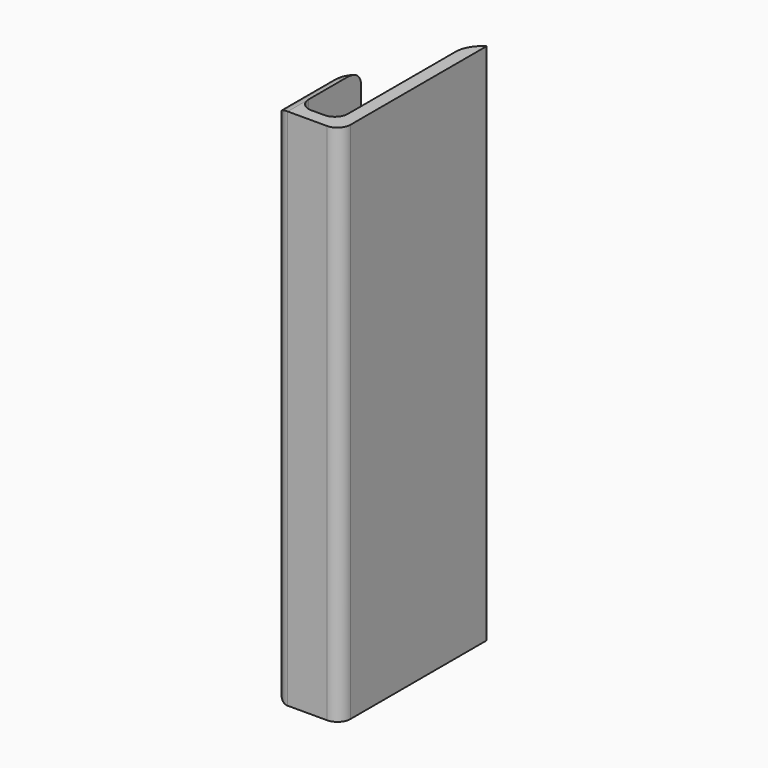
from build123d import *

# Parameters (mm, degrees)
F1_DEPTH    = 40
F2_T1_DEPTH = 48.6602540378
F3_R        = 0.99999


# Not quite as in the source:
# - a fillet or chamfer that OpenCascade refuses, or shapes differently, is made with other operations: its cross-section is extruded or revolved along the edge and cut away or added
# - a fillet or chamfer is up to 0.001 mm smaller than in the source, because OpenCascade refuses the exact size


with BuildPart() as f1:
    # F0 (on Top) → F1 (new body)
    with BuildSketch(Plane.XY):
        Polygon((-5, 0), (0, 0), (0, 14), (-1, 14), (-1, 1), (-4, 1), (-4, 7), (-5, 7), align=None)
    extrude(amount=F1_DEPTH)

    # F2: fillet of radius 2 on 2 edges, made by hand

    # F2_s2 → F2_t1 (cut)
    with BuildSketch(Plane.XY.offset(-4.3301270189)):
        with BuildLine():
            ThreePointArc((-4, 7), (-4.7320508076, 6.2679491924), (-5, 5.2679491924))
            Line((-5, 5.2679491924), (-5, 7))
            Line((-5, 7), (-4, 7))
        make_face()
        with BuildLine():
            ThreePointArc((0, 14), (-0.7320508076, 13.2679491924), (-1, 12.2679491924))
            Line((-1, 12.2679491924), (-1, 14))
            Line((-1, 14), (0, 14))
        make_face()
    extrude(amount=F2_T1_DEPTH, mode=Mode.SUBTRACT)

    # F3 (radius 1 in the source; OpenCascade refuses exactly that, so slightly less here)
    f3_edges = [f1.edges().sort_by_distance(p)[0] for p in [
        (-5, 2.633975, 40),
        (-5, 2.633975, 0),
        (-5, 0, 20),
        (0, 0, 20),
        (-4, 1, 20),
        (-1, 1, 20),
        (-4.732051, 6.267949, 0),
        (-4.732051, 6.267949, 40),
    ]]
    fillet(f3_edges, radius=F3_R)


solid = f1.part
